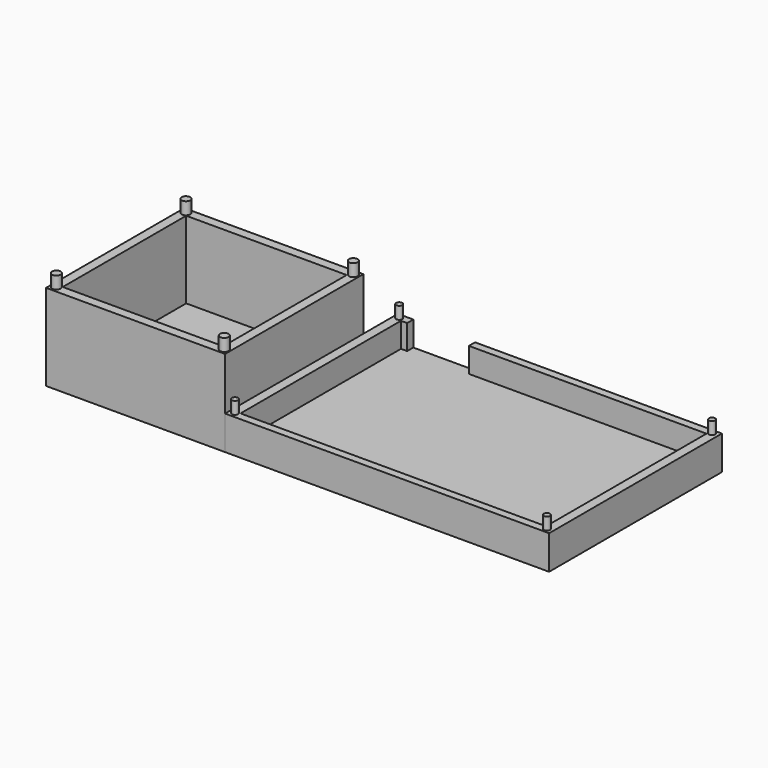
from build123d import *

# Parameters (mm, degrees)
F1_W      = 58
F1_H      = 56
F2_DEPTH  = 11
F0_W      = 105
F0_H      = 70
F3_W      = 99
F3_H      = 65
F4_DEPTH  = 8
F5_W      = 20
F5_H      = 8
F6_DEPTH  = 2.5
F7_W      = 52
F7_H      = 50
F8_DEPTH  = 8
F9_R      = 4
F10_DEPTH = 4
F11_DEPTH = 17
F12_R     = 2.5
F13_DEPTH = 3
F14_R     = 1.4
F15_DEPTH = 4
F16_R     = 1.4
F17_DEPTH = 4
F18_R     = 1
F19_DEPTH = 4
F20_R     = 1
F21_DEPTH = 4
F22_R     = 1
F23_DEPTH = 4
F24_R     = 1
F25_DEPTH = 4


with BuildPart() as f2:
    # F1 (on Top) → F2 (new body)
    with BuildSketch(Plane.XY):
        with Locations((-81.5, -7)):
            Rectangle(F1_W, F1_H)
    extrude(amount=F2_DEPTH)

    # F7 (on face) → F8 (cut)
    with BuildSketch(Plane.XY.offset(11)):
        with Locations((-81.5, -7)):
            Rectangle(F7_W, F7_H)
    extrude(amount=-F8_DEPTH, mode=Mode.SUBTRACT)

    # F9 (on face) → F10 (cut)
    with BuildSketch(Plane(origin=(0, 0, 0), x_dir=(1, 0, 0), z_dir=(0, 0, -1))):
        with Locations((-100.399762392, 19.4988027215)):
            Circle(F9_R)
    extrude(amount=-F10_DEPTH, mode=Mode.SUBTRACT)

    # F11 (add): a face of the model
    f11_faces = [f2.faces().sort_by_distance(p)[0] for p in [
        (-53.3062257748, -7, 11),
    ]]
    extrude(f11_faces, amount=F11_DEPTH)

    # F12 (on face) → F13 (cut)
    with BuildSketch(Plane(origin=(0, 21, 0), x_dir=(-1, 0, 0), z_dir=(0, 1, 0))):
        with Locations((57.8828938305, 6.8415487185)):
            Circle(F12_R)
    extrude(amount=-F13_DEPTH, mode=Mode.SUBTRACT)

    # F14 (on face) → F15 (join)
    with BuildSketch(Plane.XY.offset(28)):
        with Locations((-108.5691526532, 19.2284081131)):
            Circle(F14_R)
    extrude(amount=F15_DEPTH)

    # F16 (on face) → F17 (join)
    with BuildSketch(Plane.XY.offset(28)):
        with Locations((-108.75300318, -33.0420061946)):
            Circle(F16_R)
        with Locations((-54.1975349188, -33.2027859986)):
            Circle(F16_R)
        with Locations((-54.2859174311, 19.2066654563)):
            Circle(F16_R)
    extrude(amount=F17_DEPTH)


with BuildPart() as f2b:
    # F0 (on Top) → F2, piece 2 (new body)
    with BuildSketch(Plane.XY):
        Rectangle(F0_W, F0_H)
    extrude(amount=F2_DEPTH)

    # F3 (on face) → F4 (cut)
    with BuildSketch(Plane.XY.offset(11)):
        Rectangle(F3_W, F3_H)
    extrude(amount=-F4_DEPTH, mode=Mode.SUBTRACT)

    # F5 (on face) → F6 (cut)
    with BuildSketch(Plane(origin=(0, 35, 0), x_dir=(-1, 0, 0), z_dir=(0, 1, 0))):
        with Locations((37.5, 7)):
            Rectangle(F5_W, F5_H)
    extrude(amount=-F6_DEPTH, mode=Mode.SUBTRACT)

    # F18 (on face) → F19 (join)
    with BuildSketch(Plane.XY.offset(11)):
        with Locations((-50.7920049131, 33.3879701793)):
            Circle(F18_R)
    extrude(amount=F19_DEPTH)

    # F20 (on face) → F21 (join)
    with BuildSketch(Plane.XY.offset(11)):
        with Locations((50.4908375442, 33.5)):
            Circle(F20_R)
    extrude(amount=F21_DEPTH)

    # F22 (on face) → F23 (join)
    with BuildSketch(Plane.XY.offset(11)):
        with Locations((50.5457408726, -33.4684327245)):
            Circle(F22_R)
    extrude(amount=F23_DEPTH)

    # F24 (on face) → F25 (join)
    with BuildSketch(Plane.XY.offset(11)):
        with Locations((-50.7011041045, -33.2145504653)):
            Circle(F24_R)
    extrude(amount=F25_DEPTH)


solid = Compound([f2.part, f2b.part])
